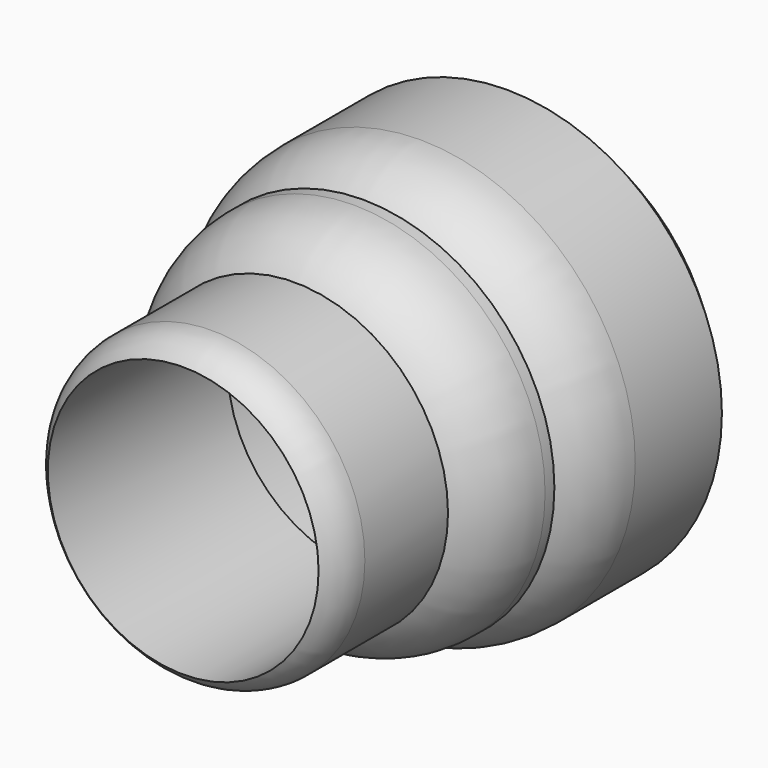
from build123d import *

# Parameters (mm, degrees)
F0_R     = 12.15
F0_R_2   = 10.15
F1_DEPTH = 15.24
F2_R     = 8.65
F2_R_2   = 7.65
F3_DEPTH = 12.7
F4_R     = 10.8128537481
F4_R_2   = 8.2306905139
F5_DEPTH = 5.08


# Not quite as in the source:
# - a fillet or chamfer that OpenCascade refuses, or shapes differently, is made with other operations: its cross-section is extruded or revolved along the edge and cut away or added


with BuildPart() as f1:
    # F0 (on Front) → F1 (new body)
    with BuildSketch(Plane.XZ):
        Circle(F0_R)
        Circle(F0_R_2, mode=Mode.SUBTRACT)
    extrude(amount=F1_DEPTH)

    # F6: fillet of radius 5.08 on 1 edges, made by hand

    # F6_s1 → F6_t2 (revolve, cut)
    with BuildSketch(Plane.XY):
        with BuildLine():
            ThreePointArc((12.15, -11.2001980247), (11.6226256161, -13.4540835586), (10.15, -15.24))
            Line((10.15, -15.24), (12.15, -15.24))
            Line((12.15, -15.24), (12.15, -11.2001980247))
        make_face()
    revolve(axis=Axis((0, -15.24, 0), (0, -1, 0)), mode=Mode.SUBTRACT)

    # F9: chamfer of 5.08 on 1 edges, made by hand

    # F9_s1 → F9_t2 (revolve, cut)
    with BuildSketch(Plane.XY):
        Polygon((12.15, -5.08), (7.07, 0), (12.15, 0), align=None)
    revolve(axis=Axis((0, 0, 0), (0, -1, 0)), mode=Mode.SUBTRACT)


with BuildPart() as f3:
    # F2 (on face) → F3 (new body)
    with BuildSketch(Plane.XZ.offset(15.24)):
        Circle(F2_R)
        Circle(F2_R_2, mode=Mode.SUBTRACT)
    extrude(amount=F3_DEPTH)

    # F8: fillet of radius 2.54 on 1 edges, made by hand

    # F8_s1 → F8_t2 (revolve, cut)
    with BuildSketch(Plane.XY):
        with BuildLine():
            ThreePointArc((8.65, -25.9200990123), (8.386312808, -27.0470417793), (7.65, -27.94))
            Line((7.65, -27.94), (8.65, -27.94))
            Line((8.65, -27.94), (8.65, -25.9200990123))
        make_face()
    revolve(axis=Axis((0, -27.94, 0), (0, -1, 0)), mode=Mode.SUBTRACT)


with BuildPart() as f5:
    # F4 (on face) → F5 (new body)
    with BuildSketch(Plane.XZ.offset(15.24)):
        Circle(F4_R)
        Circle(F4_R_2, mode=Mode.SUBTRACT)
    extrude(amount=F5_DEPTH)

    # F7: fillet of radius 5.08 on 1 edges, made by hand

    # F7_s1 → F7_t2 (revolve, cut)
    with BuildSketch(Plane.XY):
        with BuildLine():
            ThreePointArc((10.8128537481, -15.8965159104), (10.1200744383, -18.457510759), (8.2306905139, -20.32))
            Line((8.2306905139, -20.32), (10.8128537481, -20.32))
            Line((10.8128537481, -20.32), (10.8128537481, -15.8965159104))
        make_face()
    revolve(axis=Axis((0, -20.32, 0), (0, -1, 0)), mode=Mode.SUBTRACT)


solid = Compound([f1.part, f3.part, f5.part])
